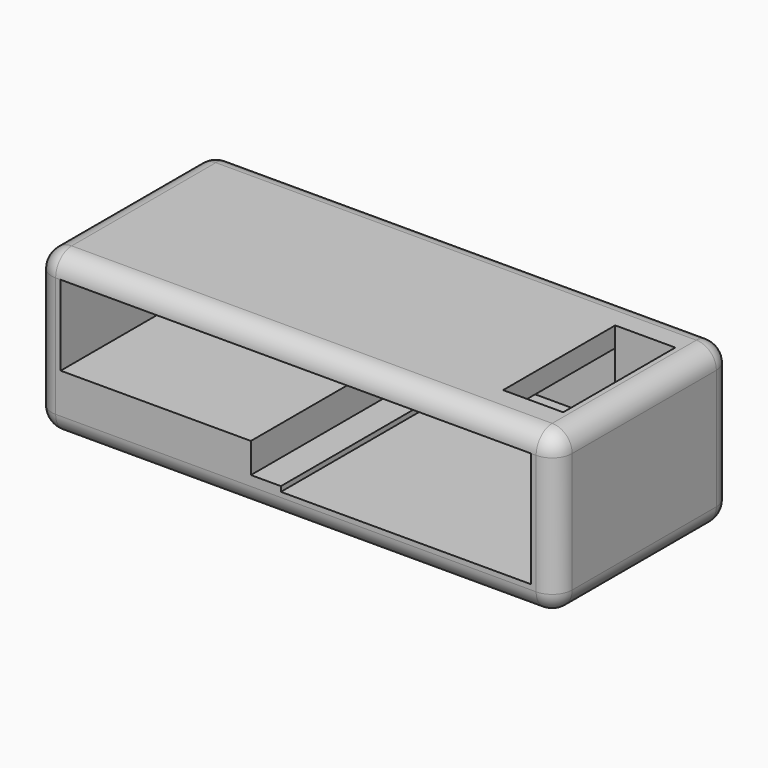
from build123d import *

# Parameters (mm, degrees)
F0_W           = 52
F0_H           = 22
F1_DEPTH       = 16
F2_W           = 41
F2_H           = 8
F3_DEPTH       = 20
F4_W           = 6
F4_H           = 10
F5_DEPTH       = 18
F6_W           = 3
F6_H           = 3
F7_DEPTH       = 22
F8_W           = 4
F8_H           = 2
F9_DEPTH       = 6
F10_T1_DEPTH   = 18
F10_T3_DEPTH   = 12
F10_T5_DEPTH   = 48
F10_T7_DEPTH   = 3
F10_T9_DEPTH   = 3
F10_S13_W      = 2
F10_S13_H      = 2
F10_T14_DEPTH  = 2
F10_S19_W      = 2
F10_S19_H      = 2
F10_T20_DEPTH  = 2
F10_S25_W      = 2
F10_S25_H      = 2
F10_T26_DEPTH  = 2
F10_S31_W      = 2
F10_S31_H      = 2
F10_T32_DEPTH  = 2
F10_S37_W      = 2
F10_S37_H      = 2
F10_T38_DEPTH  = 2
F10_S43_W      = 2
F10_S43_H      = 2
F10_T44_DEPTH  = 2
F10_S49_W      = 2
F10_S49_H      = 2
F10_T50_DEPTH  = 2
F10_S55_W      = 2
F10_S55_H      = 2
F10_T56_DEPTH  = 2
F10_T63_DEPTH  = 8
F10_T67_DEPTH  = 8
F10_T74_DEPTH  = 8
F10_T78_DEPTH  = 8
F10_T85_DEPTH  = 8
F10_T89_DEPTH  = 8
F10_T96_DEPTH  = 8
F10_T100_DEPTH = 8


# Not quite as in the source:
# - a fillet or chamfer that OpenCascade refuses, or shapes differently, is made with other operations: its cross-section is extruded or revolved along the edge and cut away or added


with BuildPart() as f1:
    # F0 (on Top) → F1 (new body)
    with BuildSketch(Plane.XY):
        Rectangle(F0_W, F0_H)
    extrude(amount=F1_DEPTH)

    # F2 (on face) → F3 (cut)
    with BuildSketch(Plane.XZ.offset(11)):
        with Locations((-3, 10)):
            Rectangle(F2_W, F2_H)
    extrude(amount=-F3_DEPTH, mode=Mode.SUBTRACT)

    # F4 (on face) → F5 (cut)
    with BuildSketch(Plane.XZ.offset(11)):
        Polygon((17.5, 6), (-1.5, 6), (-1.5, 2.5), (23.5, 2.5), (23.5, 6), align=None)
        with Locations((20.5, 11)):
            Rectangle(F4_W, F4_H)
    extrude(amount=-F5_DEPTH, mode=Mode.SUBTRACT)

    # F6 (on face) → F7 (cut, through all)
    with BuildSketch(Plane.XZ.offset(11)):
        with Locations((-3, 4.5)):
            Rectangle(F6_W, F6_H)
    extrude(amount=-F7_DEPTH, mode=Mode.SUBTRACT)

    # F8 (on face) → F9 (join)
    with BuildSketch(Plane(origin=(23.5, 0, 0), x_dir=(0, -1, 0), z_dir=(-1, 0, 0))):
        with Locations((9, 15)):
            Rectangle(F8_W, F8_H)
    extrude(amount=F9_DEPTH)

    # F10: fillet of radius 2 on 16 edges, made by hand

    # F10_s2 → F10_t1 (cut)
    with BuildSketch(Plane.XZ.offset(-9)):
        with BuildLine():
            ThreePointArc((-26, 2), (-25.4142135624, 0.5857864376), (-24, 0))
            Line((-24, 0), (-26, 0))
            Line((-26, 0), (-26, 2))
        make_face()
        with BuildLine():
            ThreePointArc((-24, 16), (-25.4142135624, 15.4142135624), (-26, 14))
            Line((-26, 14), (-26, 16))
            Line((-26, 16), (-24, 16))
        make_face()
        with BuildLine():
            ThreePointArc((26, 14), (25.4142135624, 15.4142135624), (24, 16))
            Line((24, 16), (26, 16))
            Line((26, 16), (26, 14))
        make_face()
        with BuildLine():
            ThreePointArc((26, 2), (25.4142135624, 0.5857864376), (24, 0))
            Line((24, 0), (26, 0))
            Line((26, 0), (26, 2))
        make_face()
    extrude(amount=F10_T1_DEPTH, mode=Mode.SUBTRACT)

    # F10_s4 → F10_t3 (cut)
    with BuildSketch(Plane.XY.offset(2)):
        with BuildLine():
            ThreePointArc((-24, -11), (-25.4142135624, -10.4142135624), (-26, -9))
            Line((-26, -9), (-26, -11))
            Line((-26, -11), (-24, -11))
        make_face()
        with BuildLine():
            ThreePointArc((24, -11), (25.4142135624, -10.4142135624), (26, -9))
            Line((26, -9), (26, -11))
            Line((26, -11), (24, -11))
        make_face()
        with BuildLine():
            ThreePointArc((24, 11), (25.4142135624, 10.4142135624), (26, 9))
            Line((26, 9), (26, 11))
            Line((26, 11), (24, 11))
        make_face()
        with BuildLine():
            ThreePointArc((-24, 11), (-25.4142135624, 10.4142135624), (-26, 9))
            Line((-26, 9), (-26, 11))
            Line((-26, 11), (-24, 11))
        make_face()
    extrude(amount=F10_T3_DEPTH, mode=Mode.SUBTRACT)

    # F10_s6 → F10_t5 (cut)
    with BuildSketch(Plane.YZ.offset(-24)):
        with BuildLine():
            ThreePointArc((-11, 14), (-10.4142135624, 15.4142135624), (-9, 16))
            Line((-9, 16), (-11, 16))
            Line((-11, 16), (-11, 14))
        make_face()
        with BuildLine():
            ThreePointArc((-11, 2), (-10.4142135624, 0.5857864376), (-9, 0))
            Line((-9, 0), (-11, 0))
            Line((-11, 0), (-11, 2))
        make_face()
        with BuildLine():
            ThreePointArc((11, 14), (10.4142135624, 15.4142135624), (9, 16))
            Line((9, 16), (11, 16))
            Line((11, 16), (11, 14))
        make_face()
        with BuildLine():
            ThreePointArc((11, 2), (10.4142135624, 0.5857864376), (9, 0))
            Line((9, 0), (11, 0))
            Line((11, 0), (11, 2))
        make_face()
    extrude(amount=F10_T5_DEPTH, mode=Mode.SUBTRACT)

    # F10_s8 → F10_t7 (cut)
    with BuildSketch(Plane.YZ.offset(-4.5)):
        with BuildLine():
            ThreePointArc((9, 6), (10.4142135624, 6.5857864376), (11, 8))
            Line((11, 8), (11, 6))
            Line((11, 6), (9, 6))
        make_face()
        with BuildLine():
            ThreePointArc((11, 1), (10.4142135624, 2.4142135624), (9, 3))
            Line((9, 3), (11, 3))
            Line((11, 3), (11, 1))
        make_face()
    extrude(amount=F10_T7_DEPTH, mode=Mode.SUBTRACT)

    # F10_s10 → F10_t9 (cut)
    with BuildSketch(Plane.XY.offset(3)):
        with BuildLine():
            ThreePointArc((-6.5, 11), (-5.0857864376, 10.4142135624), (-4.5, 9))
            Line((-4.5, 9), (-4.5, 11))
            Line((-4.5, 11), (-6.5, 11))
        make_face()
        with BuildLine():
            ThreePointArc((0.5, 11), (-0.9142135624, 10.4142135624), (-1.5, 9))
            Line((-1.5, 9), (-1.5, 11))
            Line((-1.5, 11), (0.5, 11))
        make_face()
    extrude(amount=F10_T9_DEPTH, mode=Mode.SUBTRACT)


with BuildPart() as f10_tool12:
    # F10_s13 → F10_t14 (new body)
    with BuildSketch(Plane.YZ.offset(-24)):
        with Locations((10, 1)):
            Rectangle(F10_S13_W, F10_S13_H)
    extrude(amount=-F10_T14_DEPTH)

    # F10_s15 → F10_t16 (revolve, cut)
    with BuildSketch(Plane(origin=(-24, 9, 2), x_dir=(0, -0.7071067812, 0.7071067812), z_dir=(0, -0.7071067812, -0.7071067812))):
        with BuildLine():
            ThreePointArc((0, -2), (2, 0), (0, 2))
            Line((0, 2), (0, -2))
        make_face()
    revolve(axis=Axis((-24, 9, 2), (-1, 0, 0)), mode=Mode.SUBTRACT)


with BuildPart() as f1_1:
    add(f1.part)

    # F10_t11: cut F10_tool12
    add(f10_tool12.part, mode=Mode.SUBTRACT)


with BuildPart() as f10_tool18:
    # F10_s19 → F10_t20 (new body)
    with BuildSketch(Plane.XZ.offset(9)):
        with Locations((-25, 1)):
            Rectangle(F10_S19_W, F10_S19_H)
    extrude(amount=F10_T20_DEPTH)

    # F10_s21 → F10_t22 (revolve, cut)
    with BuildSketch(Plane(origin=(-24, -9, 2), x_dir=(0.7071067812, 0, 0.7071067812), z_dir=(0.7071067812, 0, -0.7071067812))):
        with BuildLine():
            ThreePointArc((0, -2), (2, 0), (0, 2))
            Line((0, 2), (0, -2))
        make_face()
    revolve(axis=Axis((-24, -9, 2), (0, -1, 0)), mode=Mode.SUBTRACT)


with BuildPart() as f1_2:
    add(f1_1.part)

    # F10_t17: cut F10_tool18
    add(f10_tool18.part, mode=Mode.SUBTRACT)


with BuildPart() as f10_tool24:
    # F10_s25 → F10_t26 (new body)
    with BuildSketch(Plane.XZ.offset(9)):
        with Locations((-25, 15)):
            Rectangle(F10_S25_W, F10_S25_H)
    extrude(amount=F10_T26_DEPTH)

    # F10_s27 → F10_t28 (revolve, cut)
    with BuildSketch(Plane(origin=(-24, -9, 14), x_dir=(0.7071067812, 0, -0.7071067812), z_dir=(-0.7071067812, 0, -0.7071067812))):
        with BuildLine():
            ThreePointArc((0, -2), (2, 0), (0, 2))
            Line((0, 2), (0, -2))
        make_face()
    revolve(axis=Axis((-24, -9, 14), (0, -1, 0)), mode=Mode.SUBTRACT)


with BuildPart() as f1_3:
    add(f1_2.part)

    # F10_t23: cut F10_tool24
    add(f10_tool24.part, mode=Mode.SUBTRACT)


with BuildPart() as f10_tool30:
    # F10_s31 → F10_t32 (new body)
    with BuildSketch(Plane.XZ.offset(9)):
        with Locations((25, 15)):
            Rectangle(F10_S31_W, F10_S31_H)
    extrude(amount=F10_T32_DEPTH)

    # F10_s33 → F10_t34 (revolve, cut)
    with BuildSketch(Plane(origin=(24, -9, 14), x_dir=(-0.7071067812, 0, -0.7071067812), z_dir=(-0.7071067812, 0, 0.7071067812))):
        with BuildLine():
            ThreePointArc((0, -2), (2, 0), (0, 2))
            Line((0, 2), (0, -2))
        make_face()
    revolve(axis=Axis((24, -9, 14), (0, -1, 0)), mode=Mode.SUBTRACT)


with BuildPart() as f1_4:
    add(f1_3.part)

    # F10_t29: cut F10_tool30
    add(f10_tool30.part, mode=Mode.SUBTRACT)


with BuildPart() as f10_tool36:
    # F10_s37 → F10_t38 (new body)
    with BuildSketch(Plane.XY.offset(14)):
        with Locations((-25, 10)):
            Rectangle(F10_S37_W, F10_S37_H)
    extrude(amount=F10_T38_DEPTH)

    # F10_s39 → F10_t40 (revolve, cut)
    with BuildSketch(Plane(origin=(-24, 9, 14), x_dir=(0.7071067812, -0.7071067812, 0), z_dir=(-0.7071067812, -0.7071067812, 0))):
        with BuildLine():
            ThreePointArc((0, -2), (2, 0), (0, 2))
            Line((0, 2), (0, -2))
        make_face()
    revolve(axis=Axis((-24, 9, 14), (0, 0, 1)), mode=Mode.SUBTRACT)


with BuildPart() as f1_5:
    add(f1_4.part)

    # F10_t35: cut F10_tool36
    add(f10_tool36.part, mode=Mode.SUBTRACT)


with BuildPart() as f10_tool42:
    # F10_s43 → F10_t44 (new body)
    with BuildSketch(Plane.XZ.offset(9)):
        with Locations((25, 1)):
            Rectangle(F10_S43_W, F10_S43_H)
    extrude(amount=F10_T44_DEPTH)

    # F10_s45 → F10_t46 (revolve, cut)
    with BuildSketch(Plane(origin=(24, -9, 2), x_dir=(-0.7071067812, 0, 0.7071067812), z_dir=(0.7071067812, 0, 0.7071067812))):
        with BuildLine():
            ThreePointArc((0, -2), (2, 0), (0, 2))
            Line((0, 2), (0, -2))
        make_face()
    revolve(axis=Axis((24, -9, 2), (0, -1, 0)), mode=Mode.SUBTRACT)


with BuildPart() as f1_6:
    add(f1_5.part)

    # F10_t41: cut F10_tool42
    add(f10_tool42.part, mode=Mode.SUBTRACT)


with BuildPart() as f10_tool48:
    # F10_s49 → F10_t50 (new body)
    with BuildSketch(Plane.YZ.offset(24)):
        with Locations((10, 15)):
            Rectangle(F10_S49_W, F10_S49_H)
    extrude(amount=F10_T50_DEPTH)

    # F10_s51 → F10_t52 (revolve, cut)
    with BuildSketch(Plane(origin=(24, 9, 14), x_dir=(0, -0.7071067812, -0.7071067812), z_dir=(0, -0.7071067812, 0.7071067812))):
        with BuildLine():
            ThreePointArc((0, -2), (2, 0), (0, 2))
            Line((0, 2), (0, -2))
        make_face()
    revolve(axis=Axis((24, 9, 14), (1, 0, 0)), mode=Mode.SUBTRACT)


with BuildPart() as f1_7:
    add(f1_6.part)

    # F10_t47: cut F10_tool48
    add(f10_tool48.part, mode=Mode.SUBTRACT)


with BuildPart() as f10_tool54:
    # F10_s55 → F10_t56 (new body)
    with BuildSketch(Plane.YZ.offset(24)):
        with Locations((10, 1)):
            Rectangle(F10_S55_W, F10_S55_H)
    extrude(amount=F10_T56_DEPTH)

    # F10_s57 → F10_t58 (revolve, cut)
    with BuildSketch(Plane(origin=(24, 9, 2), x_dir=(0, -0.7071067812, 0.7071067812), z_dir=(0, 0.7071067812, 0.7071067812))):
        with BuildLine():
            ThreePointArc((0, -2), (2, 0), (0, 2))
            Line((0, 2), (0, -2))
        make_face()
    revolve(axis=Axis((24, 9, 2), (1, 0, 0)), mode=Mode.SUBTRACT)


with BuildPart() as f1_8:
    add(f1_7.part)

    # F10_t53: cut F10_tool54
    add(f10_tool54.part, mode=Mode.SUBTRACT)


with BuildPart() as f10_tool61:
    # F10_s62 → F10_t63 (new body)
    with BuildSketch(Plane.YZ.offset(3.5)):
        with BuildLine():
            ThreePointArc((9, 6), (10.4142135624, 6.5857864376), (11, 8))
            Line((11, 8), (11, 6))
            Line((11, 6), (9, 6))
        make_face()
    extrude(amount=-F10_T63_DEPTH)

    split(bisect_by=Plane.YZ.offset(-1.5), keep=Keep.TOP)


with BuildPart() as f10_tool65:
    # F10_s66 → F10_t67 (new body)
    with BuildSketch(Plane.XY.offset(3)):
        with BuildLine():
            ThreePointArc((0.5, 11), (-0.9142135624, 10.4142135624), (-1.5, 9))
            Line((-1.5, 9), (-1.5, 11))
            Line((-1.5, 11), (0.5, 11))
        make_face()
    extrude(amount=F10_T67_DEPTH)

    split(bisect_by=Plane.XY.offset(6), keep=Keep.TOP)


with BuildPart() as f10_tool61_1:
    add(f10_tool61.part)

    # F10_t69: intersect F10_tool65
    add(f10_tool65.part, mode=Mode.INTERSECT)


with BuildPart() as f1_9:
    add(f1_8.part)

    # F10_t59: cut F10_tool61
    add(f10_tool61_1.part, mode=Mode.SUBTRACT)


with BuildPart() as f10_tool72:
    # F10_s73 → F10_t74 (new body)
    with BuildSketch(Plane.YZ.offset(-1.5)):
        with BuildLine():
            ThreePointArc((9, 6), (10.4142135624, 6.5857864376), (11, 8))
            Line((11, 8), (11, 6))
            Line((11, 6), (9, 6))
        make_face()
    extrude(amount=-F10_T74_DEPTH)

    split(bisect_by=Plane.YZ.offset(-4.5), keep=Keep.BOTTOM)


with BuildPart() as f10_tool76:
    # F10_s77 → F10_t78 (new body)
    with BuildSketch(Plane.XY.offset(11)):
        with BuildLine():
            ThreePointArc((-6.5, 11), (-5.0857864376, 10.4142135624), (-4.5, 9))
            Line((-4.5, 9), (-4.5, 11))
            Line((-4.5, 11), (-6.5, 11))
        make_face()
    extrude(amount=-F10_T78_DEPTH)

    split(bisect_by=Plane.XY.offset(6), keep=Keep.TOP)


with BuildPart() as f10_tool72_1:
    add(f10_tool72.part)

    # F10_t80: intersect F10_tool76
    add(f10_tool76.part, mode=Mode.INTERSECT)


with BuildPart() as f1_10:
    add(f1_9.part)

    # F10_t70: cut F10_tool72
    add(f10_tool72_1.part, mode=Mode.SUBTRACT)


with BuildPart() as f10_tool83:
    # F10_s84 → F10_t85 (new body)
    with BuildSketch(Plane.XY.offset(6)):
        with BuildLine():
            ThreePointArc((-6.5, 11), (-5.0857864376, 10.4142135624), (-4.5, 9))
            Line((-4.5, 9), (-4.5, 11))
            Line((-4.5, 11), (-6.5, 11))
        make_face()
    extrude(amount=-F10_T85_DEPTH)

    split(bisect_by=Plane.XY.offset(3), keep=Keep.BOTTOM)


with BuildPart() as f10_tool87:
    # F10_s88 → F10_t89 (new body)
    with BuildSketch(Plane.YZ.offset(-9.5)):
        with BuildLine():
            ThreePointArc((11, 1), (10.4142135624, 2.4142135624), (9, 3))
            Line((9, 3), (11, 3))
            Line((11, 3), (11, 1))
        make_face()
    extrude(amount=F10_T89_DEPTH)

    split(bisect_by=Plane.YZ.offset(-4.5), keep=Keep.BOTTOM)


with BuildPart() as f10_tool83_1:
    add(f10_tool83.part)

    # F10_t91: intersect F10_tool87
    add(f10_tool87.part, mode=Mode.INTERSECT)


with BuildPart() as f1_11:
    add(f1_10.part)

    # F10_t81: cut F10_tool83
    add(f10_tool83_1.part, mode=Mode.SUBTRACT)


with BuildPart() as f10_tool94:
    # F10_s95 → F10_t96 (new body)
    with BuildSketch(Plane.XY.offset(-2)):
        with BuildLine():
            ThreePointArc((0.5, 11), (-0.9142135624, 10.4142135624), (-1.5, 9))
            Line((-1.5, 9), (-1.5, 11))
            Line((-1.5, 11), (0.5, 11))
        make_face()
    extrude(amount=F10_T96_DEPTH)

    split(bisect_by=Plane.XY.offset(3), keep=Keep.BOTTOM)


with BuildPart() as f10_tool98:
    # F10_s99 → F10_t100 (new body)
    with BuildSketch(Plane.YZ.offset(-4.5)):
        with BuildLine():
            ThreePointArc((11, 1), (10.4142135624, 2.4142135624), (9, 3))
            Line((9, 3), (11, 3))
            Line((11, 3), (11, 1))
        make_face()
    extrude(amount=F10_T100_DEPTH)

    split(bisect_by=Plane.YZ.offset(-1.5), keep=Keep.TOP)


with BuildPart() as f10_tool94_1:
    add(f10_tool94.part)

    # F10_t102: intersect F10_tool98
    add(f10_tool98.part, mode=Mode.INTERSECT)


with BuildPart() as f1_12:
    add(f1_11.part)

    # F10_t92: cut F10_tool94
    add(f10_tool94_1.part, mode=Mode.SUBTRACT)


solid = f1_12.part
